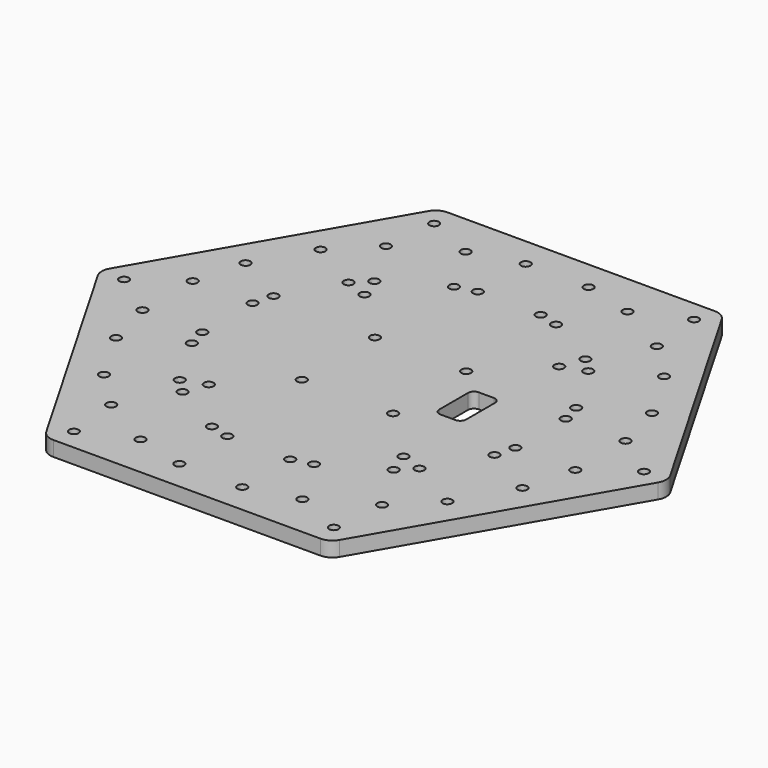
from build123d import *

# Parameters (mm, degrees)
F0_R     = 1.6
F0_R_2   = 1.575
F0_R_3   = 1.15
F0_R_4   = 5
F1_DEPTH = 5


with BuildPart() as f1:
    # F0 (on Top) → F1 (new body)
    with BuildSketch(Plane.XY):
        with BuildLine():
            Line((-93.5566243293, -2.4999999943), (-48.9433756768, -79.7724133547))
            ThreePointArc((-48.9433756768, -79.7724133547), (-47.1132486579, -81.6025403736), (-44.6132486579, -82.2724133548))
            Line((-44.6132486579, -82.2724133548), (44.6132486502, -82.2724133566))
            ThreePointArc((44.6132486502, -82.2724133566), (47.1132486502, -81.6025403755), (48.9433756692, -79.7724133566))
            Line((48.9433756692, -79.7724133566), (93.5566243248, -2.499999998))
            ThreePointArc((93.5566243248, -2.499999998), (94.2264973059, 2e-09), (93.5566243249, 2.500000002))
            Line((93.5566243249, 2.500000002), (48.9433756724, 79.7724133624))
            ThreePointArc((48.9433756724, 79.7724133624), (47.1132486535, 81.6025403814), (44.6132486535, 82.2724133625))
            Line((44.6132486535, 82.2724133625), (-44.6132486546, 82.2724133643))
            ThreePointArc((-44.6132486546, 82.2724133643), (-47.1132486546, 81.6025403832), (-48.9433756736, 79.7724133644))
            Line((-48.9433756736, 79.7724133644), (-93.5566243292, 2.5000000057))
            ThreePointArc((-93.5566243292, 2.5000000057), (-94.2264973103, 5.7e-09), (-93.5566243293, -2.4999999943))
        make_face()
        with Locations((-57.3397459654, -45.229473422)):
            Circle(F0_R, mode=Mode.SUBTRACT)
        with Locations((-43.4000000039, -75.1710050514)):
            Circle(F0_R_2, mode=Mode.SUBTRACT)
        with Locations((-27.0429399416, -67.839745966)):
            Circle(F0_R, mode=Mode.SUBTRACT)
        with Locations((-10.4999999994, -72.2724133636)):
            Circle(F0_R, mode=Mode.SUBTRACT)
        with Locations((-45.229473421, -57.339745966)):
            Circle(F0_R, mode=Mode.SUBTRACT)
        with Locations((-10.4999999994, -52.2724133636)):
            Circle(F0_R, mode=Mode.SUBTRACT)
        with Locations((-17.0429399416, -50.5192378903)):
            Circle(F0_R, mode=Mode.SUBTRACT)
        with Locations((-67.8397459654, -27.0429399426)):
            Circle(F0_R, mode=Mode.SUBTRACT)
        with Locations((-72.2724133636, -10.5000000006)):
            Circle(F0_R, mode=Mode.SUBTRACT)
        with Locations((-86.8000000044, 1.9e-09)):
            Circle(F0_R_2, mode=Mode.SUBTRACT)
        with Locations((-50.5192378897, -17.0429399426)):
            Circle(F0_R, mode=Mode.SUBTRACT)
        with Locations((-52.2724133636, -10.5000000006)):
            Circle(F0_R, mode=Mode.SUBTRACT)
        with Locations((-40.0192378897, -35.229473422)):
            Circle(F0_R, mode=Mode.SUBTRACT)
        with Locations((-35.229473421, -40.0192378903)):
            Circle(F0_R, mode=Mode.SUBTRACT)
        with Locations((-32.5, -32.5)):
            Circle(F0_R, mode=Mode.SUBTRACT)
        with Locations((-6.5, -27)):
            Circle(F0_R_3, mode=Mode.SUBTRACT)
        with Locations((-15.25, -15.25)):
            Circle(F0_R, mode=Mode.SUBTRACT)
        with Locations((10.5000000006, -72.2724133636)):
            Circle(F0_R, mode=Mode.SUBTRACT)
        with Locations((43.4000000006, -75.1710050533)):
            Circle(F0_R_2, mode=Mode.SUBTRACT)
        with Locations((27.0429399426, -67.8397459654)):
            Circle(F0_R, mode=Mode.SUBTRACT)
        with Locations((10.5000000006, -52.2724133636)):
            Circle(F0_R, mode=Mode.SUBTRACT)
        with Locations((17.0429399426, -50.5192378897)):
            Circle(F0_R, mode=Mode.SUBTRACT)
        with Locations((45.229473422, -57.3397459654)):
            Circle(F0_R, mode=Mode.SUBTRACT)
        with Locations((57.339745966, -45.229473421)):
            Circle(F0_R, mode=Mode.SUBTRACT)
        with Locations((6.5, -27)):
            Circle(F0_R_3, mode=Mode.SUBTRACT)
        with Locations((35.229473422, -40.0192378897)):
            Circle(F0_R, mode=Mode.SUBTRACT)
        with Locations((32.5, -32.5)):
            Circle(F0_R, mode=Mode.SUBTRACT)
        with Locations((40.0192378903, -35.229473421)):
            Circle(F0_R, mode=Mode.SUBTRACT)
        with Locations((15.25, -15.25)):
            Circle(F0_R, mode=Mode.SUBTRACT)
        Circle(F0_R_4, mode=Mode.SUBTRACT)
        with BuildLine():
            ThreePointArc((23.25, 6), (23.8357864376, 7.4142135624), (25.25, 8))
            Line((25.25, 8), (30.25, 8))
            ThreePointArc((30.25, 8), (31.6642135624, 7.4142135624), (32.25, 6))
            Line((32.25, 6), (32.25, -6))
            ThreePointArc((32.25, -6), (31.6642135624, -7.4142135624), (30.25, -8))
            Line((30.25, -8), (25.25, -8))
            ThreePointArc((25.25, -8), (23.8357864376, -7.4142135624), (23.25, -6))
            Line((23.25, -6), (23.25, 6))
        make_face(mode=Mode.SUBTRACT)
        with Locations((67.839745966, -27.0429399416)):
            Circle(F0_R, mode=Mode.SUBTRACT)
        with Locations((50.5192378903, -17.0429399416)):
            Circle(F0_R, mode=Mode.SUBTRACT)
        with Locations((52.2724133636, -10.4999999994)):
            Circle(F0_R, mode=Mode.SUBTRACT)
        with Locations((72.2724133636, -10.4999999994)):
            Circle(F0_R, mode=Mode.SUBTRACT)
        with Locations((86.8000000044, -1.9e-09)):
            Circle(F0_R_2, mode=Mode.SUBTRACT)
        with Locations((-72.2724133636, 10.4999999994)):
            Circle(F0_R, mode=Mode.SUBTRACT)
        with Locations((-52.2724133636, 10.4999999994)):
            Circle(F0_R, mode=Mode.SUBTRACT)
        with Locations((-50.5192378903, 17.0429399416)):
            Circle(F0_R, mode=Mode.SUBTRACT)
        with Locations((-67.839745966, 27.0429399416)):
            Circle(F0_R, mode=Mode.SUBTRACT)
        with Locations((-15.25, 15.25)):
            Circle(F0_R, mode=Mode.SUBTRACT)
        with Locations((-40.0192378903, 35.229473421)):
            Circle(F0_R, mode=Mode.SUBTRACT)
        with Locations((-32.5, 32.5)):
            Circle(F0_R, mode=Mode.SUBTRACT)
        with Locations((-35.229473422, 40.0192378897)):
            Circle(F0_R, mode=Mode.SUBTRACT)
        with Locations((-6.5, 27)):
            Circle(F0_R_3, mode=Mode.SUBTRACT)
        with Locations((-57.339745966, 45.229473421)):
            Circle(F0_R, mode=Mode.SUBTRACT)
        with Locations((-45.229473422, 57.3397459654)):
            Circle(F0_R, mode=Mode.SUBTRACT)
        with Locations((-17.0429399426, 50.5192378897)):
            Circle(F0_R, mode=Mode.SUBTRACT)
        with Locations((-10.5000000006, 52.2724133636)):
            Circle(F0_R, mode=Mode.SUBTRACT)
        with Locations((-27.0429399426, 67.8397459654)):
            Circle(F0_R, mode=Mode.SUBTRACT)
        with Locations((-43.4000000006, 75.1710050533)):
            Circle(F0_R_2, mode=Mode.SUBTRACT)
        with Locations((-10.5000000006, 72.2724133636)):
            Circle(F0_R, mode=Mode.SUBTRACT)
        with Locations((15.25, 15.25)):
            Circle(F0_R, mode=Mode.SUBTRACT)
        with Locations((6.5, 27)):
            Circle(F0_R_3, mode=Mode.SUBTRACT)
        with Locations((32.5, 32.5)):
            Circle(F0_R, mode=Mode.SUBTRACT)
        with Locations((35.229473421, 40.0192378903)):
            Circle(F0_R, mode=Mode.SUBTRACT)
        with Locations((40.0192378897, 35.229473422)):
            Circle(F0_R, mode=Mode.SUBTRACT)
        with Locations((52.2724133636, 10.5000000006)):
            Circle(F0_R, mode=Mode.SUBTRACT)
        with Locations((50.5192378897, 17.0429399426)):
            Circle(F0_R, mode=Mode.SUBTRACT)
        with Locations((72.2724133636, 10.5000000006)):
            Circle(F0_R, mode=Mode.SUBTRACT)
        with Locations((67.8397459654, 27.0429399426)):
            Circle(F0_R, mode=Mode.SUBTRACT)
        with Locations((17.0429399416, 50.5192378903)):
            Circle(F0_R, mode=Mode.SUBTRACT)
        with Locations((10.4999999994, 52.2724133636)):
            Circle(F0_R, mode=Mode.SUBTRACT)
        with Locations((45.229473421, 57.339745966)):
            Circle(F0_R, mode=Mode.SUBTRACT)
        with Locations((10.4999999994, 72.2724133636)):
            Circle(F0_R, mode=Mode.SUBTRACT)
        with Locations((27.0429399416, 67.839745966)):
            Circle(F0_R, mode=Mode.SUBTRACT)
        with Locations((43.4000000039, 75.1710050514)):
            Circle(F0_R_2, mode=Mode.SUBTRACT)
        with Locations((57.3397459654, 45.229473422)):
            Circle(F0_R, mode=Mode.SUBTRACT)
        with Locations((-6.5, -27)):
            Circle(F0_R_3)
        with Locations((6.5, -27)):
            Circle(F0_R_3)
        with Locations((6.5, 27)):
            Circle(F0_R_3)
        with Locations((-6.5, 27)):
            Circle(F0_R_3)
        Circle(F0_R_4)
    extrude(amount=F1_DEPTH)


solid = f1.part
